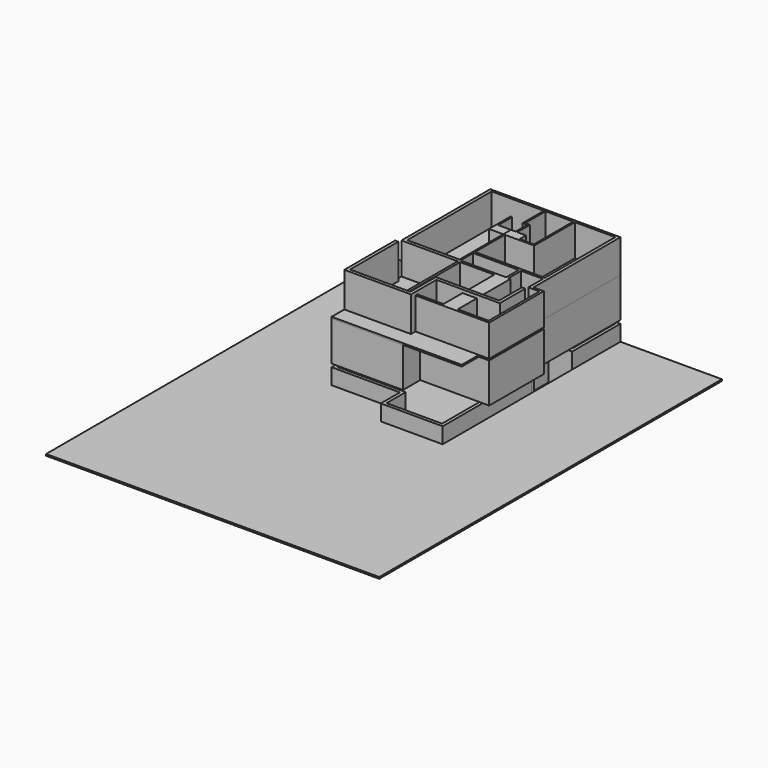
from build123d import *

# Parameters (mm, degrees)
F0_W           = 850
F0_H           = 500
F0_W_2         = 100
F0_H_2         = 3300
F0_H_3         = 1900
F0_W_3         = 1200
F0_H_4         = 100
F1_DEPTH       = 2500
F3_W           = 3700
F3_H           = 2500
F4_DEPTH       = 100
F6_W           = 8200
F6_H           = 8700
F6_W_2         = 2000
F6_H_2         = 1700
F7_DEPTH       = 100
F8_W           = 450
F8_H           = 2300
F8_W_2         = 150
F8_H_2         = 1000
F8_W_3         = 100
F8_H_3         = 900
F9_DEPTH       = 2000
F11_W          = 4100
F11_H          = 200
F11_W_2        = 100
F11_H_2        = 3300
F11_W_3        = 1100
F11_H_3        = 800
F12_DEPTH      = 2200
F8_W_4         = 1000
F8_H_4         = 600
F13_DEPTH      = 1000
F13_DEPTH_BACK = 25
F15_DEPTH      = 2200
F17_DEPTH      = 2500
F18_W          = 8200
F18_H          = 3800
F19_DEPTH      = 100
F20_W          = 200
F20_H          = 1200
F21_DEPTH      = 2200
F22_DEPTH      = 2200
F25_DEPTH      = 100


with BuildPart() as f1:
    # F0 (on Top) → F1 (new body)
    with BuildSketch(Plane.XY):
        Polygon((-4100, 4250), (-4100, -4250), (-550, -4250), (-400, -4250), (400, -4250), (400, -2750), (4100, -2750), (4100, -2600), (4100, 4250), align=None)
        Polygon((250, -4100), (-3950, -4100), (-3950, 700), (-3950, 800), (-3950, 3200), (-3950, 3300), (-3950, 4100), (-2750, 4100), (-2650, 4100), (-1650, 4100), (-1550, 4100), (-650, 4100), (-550, 4100), (1800, 4100), (1900, 4100), (3900, 4100), (3900, 800), (3900, 700), (3900, -2600), (250, -2600), align=None, mode=Mode.SUBTRACT)
        Polygon((-400, -4250), (-550, -4250), (-550, -6900), (4750, -6900), (4750, -2600), (4100, -2600), (4100, -2750), (4600, -2750), (4600, -6750), (-400, -6750), align=None)
        Polygon((-3950, 800), (-3950, 700), (-650, 700), (-550, 700), (-550, 800), (-550, 1300), (-550, 2200), (-650, 2200), (-1550, 2200), (-1550, 4100), (-1650, 4100), (-1650, 2100), (-650, 2100), (-650, 800), align=None)
        Polygon((-550, 700), (-650, 700), (-650, 400), (0, -200), (300, -200), (300, 0), (300, 700), align=None)
        with Locations((-125, 1050)):
            Rectangle(F0_W, F0_H)
        Polygon((300, 800), (300, 700), (3900, 700), (3900, 800), (1900, 800), (1800, 800), align=None)
        with Locations((1850, 2450)):
            Rectangle(F0_W_2, F0_H_2)
        Polygon((-2750, 3300), (-2750, 3200), (-2750, 2100), (-2650, 2100), (-2650, 4100), (-2750, 4100), align=None)
        with Locations((-600, 3150)):
            Rectangle(F0_W_2, F0_H_3)
        with Locations((-3350, 3250)):
            Rectangle(F0_W_3, F0_H_4)
        with Locations((-125, 750)):
            Rectangle(F0_W, F0_H_4)
    extrude(amount=F1_DEPTH)


with BuildPart() as f4:
    # F3 (on offset) → F4 (new body)
    with BuildSketch(Plane(origin=(0, 0, -200), x_dir=(1, 0, 0), z_dir=(0, 0, -1))):
        with Locations((2250, 4000)):
            Rectangle(F3_W, F3_H)
    extrude(amount=-F4_DEPTH)


with BuildPart() as f7:
    # F6 (on offset) → F7 (new body)
    with BuildSketch(Plane.XY.offset(2500)):
        with Locations((0, -100)):
            Rectangle(F6_W, F6_H)
        with Locations((-1600, 3250)):
            Rectangle(F6_W_2, F6_H_2, mode=Mode.SUBTRACT)
    extrude(amount=F7_DEPTH)

    # F8 (on face) → F9 (join)
    with BuildSketch(Plane.XY.offset(2600)):
        Polygon((-4100, 4250), (-4100, -2750), (-550, -2750), (-500, -2750), (-500, -2600), (-500, -2550), (-600, -2550), (-3900, -2550), (-3900, -440), (-3900, -340), (-3900, 2400), (-3900, 2500), (-3900, 4100), (-2700, 4100), (-2600, 4100), (-600, 4100), (-500, 4100), (1250, 4100), (1350, 4100), (3900, 4100), (3900, 1000), (3900, 900), (3900, -1450), (3900, -1600), (3900, -2550), (3900, -2750), (4100, -2750), (4100, -2600), (4100, 4250), align=None)
        Polygon((-400, -4450), (-550, -4450), (-550, -6900), (4750, -6900), (4750, -2600), (4100, -2600), (4100, -2750), (4600, -2750), (4600, -6750), (2650, -6750), (2200, -6750), (1750, -6750), (-400, -6750), align=None)
        Polygon((-500, -2750), (-550, -2750), (-550, -4450), (-400, -4450), (-400, -2750), align=None)
        Polygon((-500, -2600), (-500, -2750), (-400, -2750), (1750, -2750), (1750, -2600), align=None)
        Polygon((1750, -2600), (1750, -2750), (1750, -4450), (2200, -4450), (2200, -2600), align=None)
        Polygon((2377.0678043365, -2600), (2200, -2600), (2200, -4450), (2650, -4450), (2650, -2600), (2527.0678043365, -2600), align=None)
        with Locations((1975, -5600)):
            Rectangle(F8_W, F8_H)
        with Locations((2425, -5600)):
            Rectangle(F8_W, F8_H)
        Polygon((-600, -2550), (-500, -2550), (-500, -1600), (-500, -1450), (-500, 900), (1250, 900), (1250, 1000), (350, 1000), (-600, 1000), align=None)
        Polygon((-500, -1450), (-500, -1600), (2377.0678043365, -1600), (2527.0678043365, -1600), (3900, -1600), (3900, -1450), align=None)
        with Locations((2452.0678043365, -2100)):
            Rectangle(F8_W_2, F8_H_2)
        Polygon((1250, 2400), (1250, 1000), (1250, 900), (1350, 900), (1350, 1000), (1350, 2400), align=None)
        Polygon((-600, 2400), (-500, 2400), (-500, 2500), (-500, 4100), (-600, 4100), align=None)
        with Locations((-250, 1950)):
            Rectangle(F8_W_3, F8_H_3)
        Polygon((-600, 1500), (-600, 1000), (350, 1000), (350, 1500), (-200, 1500), (-300, 1500), align=None)
        Polygon((-500, 2400), (-300, 2400), (-200, 2400), (-200, 2500), (-500, 2500), align=None)
        Polygon((1250, 2500), (1250, 2400), (1350, 2400), (1350, 4100), (1250, 4100), align=None)
    extrude(amount=F9_DEPTH)

    # F8 (on face) → F13 (join, two sides)
    with BuildSketch(Plane.XY.offset(2600)) as f13_sk:
        with Locations((-2100, 2700)):
            Rectangle(F8_W_4, F8_H_4)
        Polygon((-2700, 2500), (-2700, 2400), (-2600, 2400), (-2600, 3000), (-2600, 4100), (-2700, 4100), align=None)
    extrude(amount=F13_DEPTH)
    extrude(f13_sk.sketch, amount=-F13_DEPTH_BACK)


with BuildPart() as f12:
    # F11 (on offset) → F12 (new body)
    with BuildSketch(Plane(origin=(0, 0, -2400), x_dir=(1, 0, 0), z_dir=(0, 0, -1))):
        Polygon((-4100, 2750), (-4100, -4250), (4100, -4250), (4100, -450), (2600, -450), (2600, 2550), (2600, 2750), (400, 2750), (400, 4250), (-4100, 4250), align=None)
        Polygon((-2900, -4050), (-3900, -4050), (-3900, -2300), (-3900, -2200), (-3900, -750), (-3900, -500), (-3900, 2550), (-3900, 2750), (-3900, 4050), (200, 4050), (200, 2750), (200, 2550), (2300, 2550), (2300, -500), (2300, -750), (3900, -750), (3900, -4050), (2000, -4050), (1900, -4050), (-700, -4050), (-800, -4050), (-1700, -4050), (-1800, -4050), (-2800, -4050), align=None, mode=Mode.SUBTRACT)
        with Locations((-1850, 2650)):
            Rectangle(F11_W, F11_H)
        Polygon((-3900, -500), (-3900, -750), (-800, -750), (-700, -750), (1900, -750), (2000, -750), (2300, -750), (2300, -500), align=None)
        with Locations((1950, -2400)):
            Rectangle(F11_W_2, F11_H_2)
        Polygon((-700, -750), (-800, -750), (-800, -2200), (-800, -2300), (-800, -4050), (-700, -4050), align=None)
        Polygon((-2900, -2300), (-2900, -4050), (-2800, -4050), (-2800, -2200), (-3900, -2200), (-3900, -2300), align=None)
        Polygon((2600, 2750), (2600, 2550), (4100, 2550), (4100, 3750), (2600, 3750), align=None)
        with Locations((3350, 3150)):
            Rectangle(F11_W_3, F11_H_3, mode=Mode.SUBTRACT)
        Polygon((-1800, -2200), (-1800, -4050), (-1700, -4050), (-1700, -2300), (-800, -2300), (-800, -2200), align=None)
    extrude(amount=-F12_DEPTH)


with BuildPart() as f15:
    # F14 (on offset) → F15 (new body)
    with BuildSketch(Plane(origin=(0, 0, -2400), x_dir=(1, 0, 0), z_dir=(0, 0, -1))):
        Polygon((-4100, 8250), (-4100, 4250), (-3900, 4250), (-3900, 8050), (400, 8050), (400, 9550), (3900, 9550), (3900, 2750), (4100, 2750), (4100, 9750), (200, 9750), (200, 8250), align=None)
    extrude(amount=-F15_DEPTH)


with BuildPart() as f17:
    # F16 (on Top) → F17 (new body)
    with BuildSketch(Plane.XY):
        Polygon((-3900, -4250), (-4100, -4250), (-4100, -8250), (400, -8250), (400, -6750), (4100, -6750), (4100, -2750), (3900, -2750), (3900, -6550), (200, -6550), (200, -8050), (-3900, -8050), align=None)
    extrude(amount=F17_DEPTH)


with BuildPart() as f19:
    # F18 (on offset) → F19 (new body)
    with BuildSketch(Plane.XY.offset(2500)):
        with Locations((0, -6350)):
            Rectangle(F18_W, F18_H)
    extrude(amount=F19_DEPTH)

    # F20 (on face) → F21 (join)
    with BuildSketch(Plane.XY.offset(2600)):
        with Locations((-4000, -3850)):
            Rectangle(F20_W, F20_H)
        Polygon((-3900, -4450), (-4100, -4450), (-4100, -7250), (100, -7250), (100, -5250), (4100, -5250), (4100, -4450), (3900, -4450), (3900, -5050), (-100, -5050), (-100, -7050), (-3900, -7050), align=None)
        with Locations((4000, -3850)):
            Rectangle(F20_W, F20_H)
    extrude(amount=F21_DEPTH)


with BuildPart() as f22:
    # F20 (on face) → F22 (new body)
    with BuildSketch(Plane.XY.offset(2600)):
        with Locations((-4000, -3850)):
            Rectangle(F20_W, F20_H)
        Polygon((-3900, -4450), (-4100, -4450), (-4100, -7250), (100, -7250), (100, -5250), (4100, -5250), (4100, -4450), (3900, -4450), (3900, -5050), (-100, -5050), (-100, -7050), (-3900, -7050), align=None)
        with Locations((4000, -3850)):
            Rectangle(F20_W, F20_H)
    extrude(amount=F22_DEPTH)


with BuildPart() as f25:
    # F24 (on offset) → F25 (new body)
    with BuildSketch(Plane.XY.offset(-1300)):
        Polygon((-4100, 4250), (-10500, 4250), (-10500, -22750), (10500, -22750), (10500, 4250), (4100, 4250), (4100, -4250), (-4100, -4250), align=None)
    extrude(amount=F25_DEPTH)


solid = Compound([f1.part, f4.part, f7.part, f12.part, f15.part, f17.part, f19.part, f22.part, f25.part])
